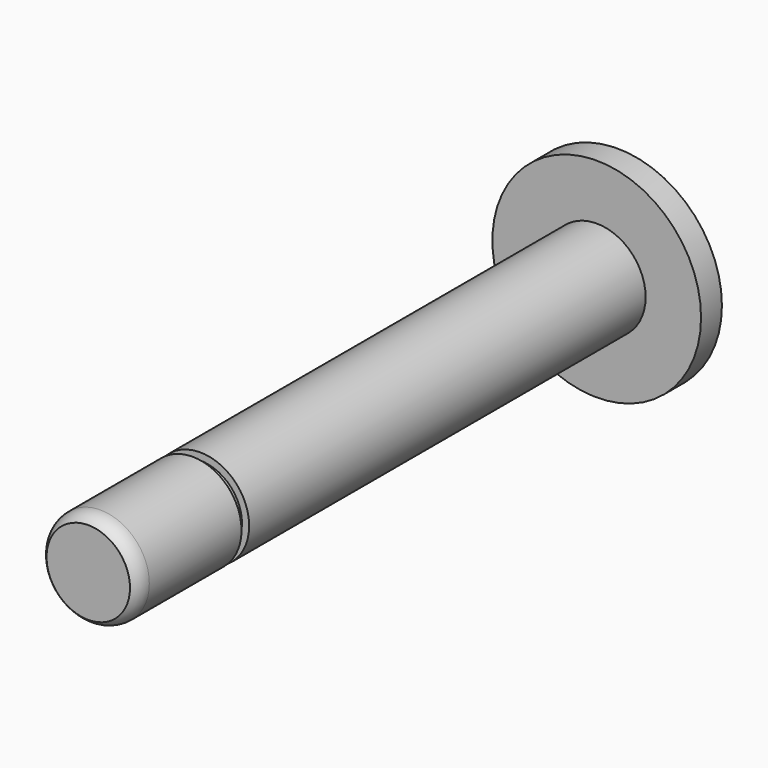
from build123d import *

# Parameters (mm, degrees)
F0_R     = 3.75
F1_DEPTH = 40
F0_R_2   = 8
F2_DEPTH = 2
F3_R     = 3.2
F4_DEPTH = 0.73
F5_R     = 3.75
F5_R_2   = 3.2
F6_DEPTH = 10
F7_DEPTH = 10


# Not quite as in the source:
# - a fillet or chamfer that OpenCascade refuses, or shapes differently, is made with other operations: its cross-section is extruded or revolved along the edge and cut away or added


with BuildPart() as f1:
    # F0 (on Front) → F1 (new body)
    with BuildSketch(Plane.XZ):
        Circle(F0_R)
    extrude(amount=F1_DEPTH)

    # F0 (on Front) → F2 (join)
    with BuildSketch(Plane.XZ):
        Circle(F0_R_2)
        Circle(F0_R, mode=Mode.SUBTRACT)
    extrude(amount=F2_DEPTH)

    # F3 (on face) → F4 (join)
    with BuildSketch(Plane.XZ.offset(40)):
        Circle(F3_R)
    extrude(amount=F4_DEPTH)


with BuildPart() as f6:
    # F5 (on face) → F6 (new body)
    with BuildSketch(Plane.XZ.offset(40.73)):
        Circle(F5_R)
        Circle(F5_R_2, mode=Mode.SUBTRACT)
    extrude(amount=F6_DEPTH)

    # F8: fillet of radius 1.5 on 1 edges, made by hand

    # F8_s1 → F8_t2 (revolve, cut)
    with BuildSketch(Plane.XY):
        with BuildLine():
            ThreePointArc((3.75, -49.5691813234), (3.6055441712, -50.2114429523), (3.2, -50.73))
            Line((3.2, -50.73), (3.75, -50.73))
            Line((3.75, -50.73), (3.75, -49.5691813234))
        make_face()
    revolve(axis=Axis((0, -50.73, 0), (0, -1, 0)), mode=Mode.SUBTRACT)


with BuildPart() as f7:
    # F7 (new): a face of the model
    f7_faces = [f1.part.faces().sort_by_distance(p)[0] for p in [
        (0, -40.73, 0),
    ]]
    extrude(f7_faces, amount=F7_DEPTH)


solid = Compound([f1.part, f6.part, f7.part])
